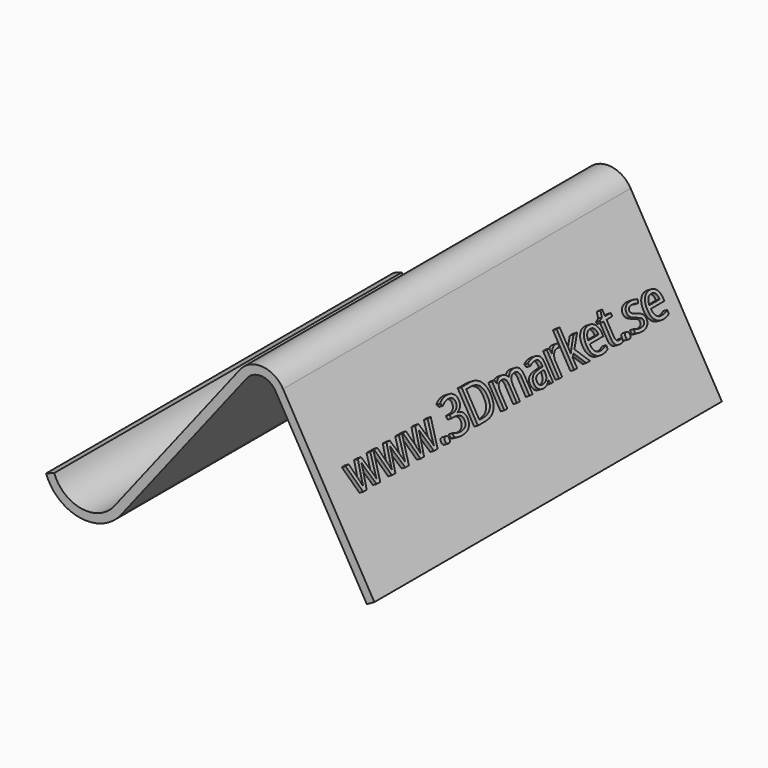
from build123d import *

# Parameters (mm, degrees)
F1_DEPTH     = 100
F2_TEXT_SIZE = 10.606172203
F3_DEPTH     = 1


# Not quite as in the source:
# - Text() gives the source's letters only with a copy of the font that has no kerning and outlines rounded to 1/6400 em; it was checked with that copy


with BuildPart() as f1:
    # F0 (on Front) → F1 (new body)
    with BuildSketch(Plane.XZ):
        with BuildLine():
            Line((23.7386193484, -1.000883263), (25.4701599035, 0))
            Line((25.4701599035, 0), (4.4516113795, 36.3623516559))
            ThreePointArc((4.4516113795, 36.3623516559), (-0.3275242067, 39.345298856), (-5.4729582171, 37.0512587965))
            Line((-5.4729582171, 37.0512587965), (-34.3901541668, 0))
            ThreePointArc((-34.3901541668, 0), (-41.9503995657, -2.9790864321), (-48.2171882592, 2.1938842745))
            Line((-48.2171882592, 2.1938842745), (-50.0972974717, 1.5118363666))
            ThreePointArc((-50.0972974717, 1.5118363666), (-42.2638116049, -4.9543770167), (-32.8135048564, -1.2305189766))
            Line((-32.8135048564, -1.2305189766), (-3.8963089066, 35.8207398199))
            ThreePointArc((-3.8963089066, 35.8207398199), (-0.4660195663, 37.3500998596), (2.7200708245, 35.3614683928))
            Line((2.7200708245, 35.3614683928), (23.7386193484, -1.000883263))
        make_face()
    extrude(amount=F1_DEPTH)

    # F2 (on face) → F3 (join)
    with BuildSketch(Plane(origin=(19.0913665344, 0, 11.0353922565), x_dir=(0, 1, 0), z_dir=(0.8657702775, 0, 0.5004416315))):
        with Locations((-94.3097574806, 5.8687630825)):
            Text('www.3Dmarket.se', F2_TEXT_SIZE, font='Open Sans', text_align=(TextAlign.LEFT, TextAlign.BOTTOM))
    extrude(amount=F3_DEPTH)


solid = f1.part
